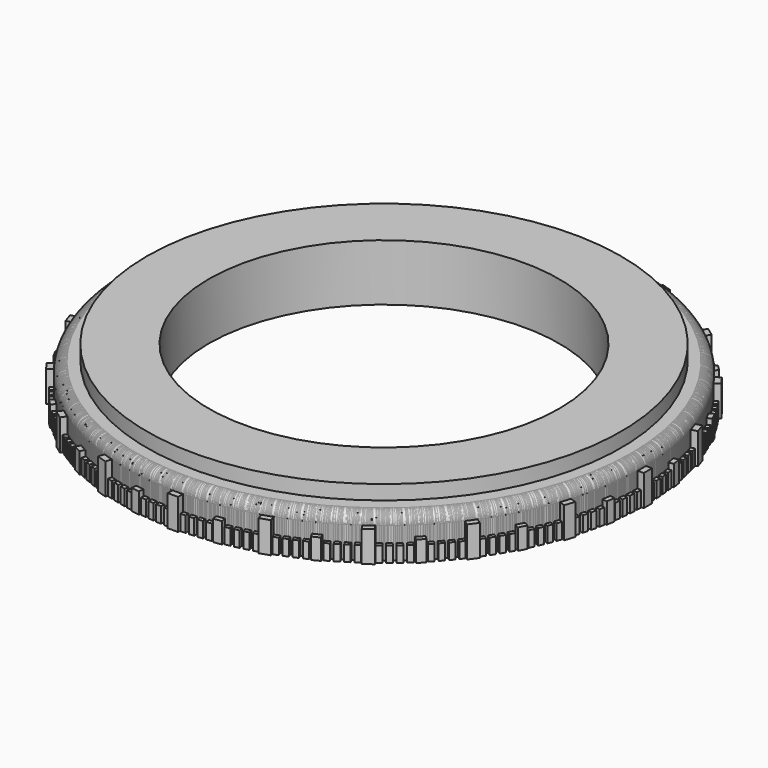
from build123d import *

# Parameters (mm, degrees)
F3_R      = 1
F4_W      = 1
F4_H      = 1
F5_DEPTH  = 3
F6_COUNT  = 20
F4_W_2    = 0.8
F4_H_2    = 0.8
F7_DEPTH  = 2
F8_COUNT  = 40
F4_W_3    = 0.5
F9_DEPTH  = 1.5
F10_COUNT = 200


with BuildPart() as f1:
    # F0 (on Front) → F1 (revolve)
    with BuildSketch(Plane.XZ):
        with BuildLine():
            Line((-20, 0), (-17, 0))
            Line((-17, 0), (-17, 4))
            Line((-17, 4), (-20, 4))
            add(Edge.make_bspline(
                [(-20, 4), (-20.2, 3.3333333333), (-20.6, 2), (-20.2, 0.6666666667), (-20, 0)],
                knots=[0, 0, 0, 0, 0.5, 1, 1, 1, 1], degree=3))
        make_face()
        Polygon((-20, 4), (-17, 4), (-17, 5.5), (-23, 5.5), (-23, 4.1), (-20, 4.1), align=None)
    revolve(axis=Axis((0, 0, 11.5319285542), (0, 0, 1)))


with BuildPart() as f2:
    # F0 (on Front) → F2 (revolve)
    with BuildSketch(Plane.XZ):
        with BuildLine():
            add(Edge.make_bspline(
                [(-20.25, 4), (-20.375, 3.3333333333), (-20.625, 2), (-20.375, 0.6666666667), (-20.25, 0)],
                knots=[0, 0, 0, 0, 0.5, 1, 1, 1, 1], degree=3))
            Line((-20.25, 4), (-25, 4))
            Line((-25, 4), (-25, 0))
            Line((-25, 0), (-20.25, 0))
        make_face()
    revolve(axis=Axis((0, 0, 11.5319285542), (0, 0, 1)))

    # F3
    f3_edges = [f2.edges().sort_by_distance(p)[0] for p in [
        (25, 0, 4),
    ]]
    fillet(f3_edges, radius=F3_R)

    # F4 (on Top) → F5 (join)
    with BuildSketch(Plane.XY):
        with Locations((-25.0881966203, 0)):
            Rectangle(F4_W, F4_H)
    extrude(amount=F5_DEPTH)


with BuildPart() as f6_1:
    # F6: instance of F2
    add(f2.part.rotate(Axis((0, 0, 11.5319285542), (0, 0, 1)), 1 * 360 / F6_COUNT))


with BuildPart() as f6_2:
    # F6: instance of F2
    add(f2.part.rotate(Axis((0, 0, 11.5319285542), (0, 0, 1)), 2 * 360 / F6_COUNT))


with BuildPart() as f6_3:
    # F6: instance of F2
    add(f2.part.rotate(Axis((0, 0, 11.5319285542), (0, 0, 1)), 3 * 360 / F6_COUNT))


with BuildPart() as f6_4:
    # F6: instance of F2
    add(f2.part.rotate(Axis((0, 0, 11.5319285542), (0, 0, 1)), 4 * 360 / F6_COUNT))


with BuildPart() as f6_5:
    # F6: instance of F2
    add(f2.part.rotate(Axis((0, 0, 11.5319285542), (0, 0, 1)), 5 * 360 / F6_COUNT))


with BuildPart() as f6_6:
    # F6: instance of F2
    add(f2.part.rotate(Axis((0, 0, 11.5319285542), (0, 0, 1)), 6 * 360 / F6_COUNT))


with BuildPart() as f6_7:
    # F6: instance of F2
    add(f2.part.rotate(Axis((0, 0, 11.5319285542), (0, 0, 1)), 7 * 360 / F6_COUNT))


with BuildPart() as f6_8:
    # F6: instance of F2
    add(f2.part.rotate(Axis((0, 0, 11.5319285542), (0, 0, 1)), 8 * 360 / F6_COUNT))


with BuildPart() as f6_9:
    # F6: instance of F2
    add(f2.part.rotate(Axis((0, 0, 11.5319285542), (0, 0, 1)), 9 * 360 / F6_COUNT))


with BuildPart() as f6_10:
    # F6: instance of F2
    add(f2.part.rotate(Axis((0, 0, 11.5319285542), (0, 0, 1)), 10 * 360 / F6_COUNT))


with BuildPart() as f6_11:
    # F6: instance of F2
    add(f2.part.rotate(Axis((0, 0, 11.5319285542), (0, 0, 1)), 11 * 360 / F6_COUNT))


with BuildPart() as f6_12:
    # F6: instance of F2
    add(f2.part.rotate(Axis((0, 0, 11.5319285542), (0, 0, 1)), 12 * 360 / F6_COUNT))


with BuildPart() as f6_13:
    # F6: instance of F2
    add(f2.part.rotate(Axis((0, 0, 11.5319285542), (0, 0, 1)), 13 * 360 / F6_COUNT))


with BuildPart() as f6_14:
    # F6: instance of F2
    add(f2.part.rotate(Axis((0, 0, 11.5319285542), (0, 0, 1)), 14 * 360 / F6_COUNT))


with BuildPart() as f6_15:
    # F6: instance of F2
    add(f2.part.rotate(Axis((0, 0, 11.5319285542), (0, 0, 1)), 15 * 360 / F6_COUNT))


with BuildPart() as f6_16:
    # F6: instance of F2
    add(f2.part.rotate(Axis((0, 0, 11.5319285542), (0, 0, 1)), 16 * 360 / F6_COUNT))


with BuildPart() as f6_17:
    # F6: instance of F2
    add(f2.part.rotate(Axis((0, 0, 11.5319285542), (0, 0, 1)), 17 * 360 / F6_COUNT))


with BuildPart() as f6_18:
    # F6: instance of F2
    add(f2.part.rotate(Axis((0, 0, 11.5319285542), (0, 0, 1)), 18 * 360 / F6_COUNT))


with BuildPart() as f6_19:
    # F6: instance of F2
    add(f2.part.rotate(Axis((0, 0, 11.5319285542), (0, 0, 1)), 19 * 360 / F6_COUNT))


with BuildPart() as f7:
    # F4 (on Top) → F7 (new body)
    with BuildSketch(Plane.XY):
        with Locations((25.0804126263, 0)):
            Rectangle(F4_W_2, F4_H_2)
    extrude(amount=F7_DEPTH)


with BuildPart() as f8_1:
    # F8: instance of F7
    add(f7.part.rotate(Axis((0, 0, 11.5319285542), (0, 0, 1)), 1 * 360 / F8_COUNT))


with BuildPart() as f8_2:
    # F8: instance of F7
    add(f7.part.rotate(Axis((0, 0, 11.5319285542), (0, 0, 1)), 2 * 360 / F8_COUNT))


with BuildPart() as f8_3:
    # F8: instance of F7
    add(f7.part.rotate(Axis((0, 0, 11.5319285542), (0, 0, 1)), 3 * 360 / F8_COUNT))


with BuildPart() as f8_4:
    # F8: instance of F7
    add(f7.part.rotate(Axis((0, 0, 11.5319285542), (0, 0, 1)), 4 * 360 / F8_COUNT))


with BuildPart() as f8_5:
    # F8: instance of F7
    add(f7.part.rotate(Axis((0, 0, 11.5319285542), (0, 0, 1)), 5 * 360 / F8_COUNT))


with BuildPart() as f8_6:
    # F8: instance of F7
    add(f7.part.rotate(Axis((0, 0, 11.5319285542), (0, 0, 1)), 6 * 360 / F8_COUNT))


with BuildPart() as f8_7:
    # F8: instance of F7
    add(f7.part.rotate(Axis((0, 0, 11.5319285542), (0, 0, 1)), 7 * 360 / F8_COUNT))


with BuildPart() as f8_8:
    # F8: instance of F7
    add(f7.part.rotate(Axis((0, 0, 11.5319285542), (0, 0, 1)), 8 * 360 / F8_COUNT))


with BuildPart() as f8_9:
    # F8: instance of F7
    add(f7.part.rotate(Axis((0, 0, 11.5319285542), (0, 0, 1)), 9 * 360 / F8_COUNT))


with BuildPart() as f8_10:
    # F8: instance of F7
    add(f7.part.rotate(Axis((0, 0, 11.5319285542), (0, 0, 1)), 10 * 360 / F8_COUNT))


with BuildPart() as f8_11:
    # F8: instance of F7
    add(f7.part.rotate(Axis((0, 0, 11.5319285542), (0, 0, 1)), 11 * 360 / F8_COUNT))


with BuildPart() as f8_12:
    # F8: instance of F7
    add(f7.part.rotate(Axis((0, 0, 11.5319285542), (0, 0, 1)), 12 * 360 / F8_COUNT))


with BuildPart() as f8_13:
    # F8: instance of F7
    add(f7.part.rotate(Axis((0, 0, 11.5319285542), (0, 0, 1)), 13 * 360 / F8_COUNT))


with BuildPart() as f8_14:
    # F8: instance of F7
    add(f7.part.rotate(Axis((0, 0, 11.5319285542), (0, 0, 1)), 14 * 360 / F8_COUNT))


with BuildPart() as f8_15:
    # F8: instance of F7
    add(f7.part.rotate(Axis((0, 0, 11.5319285542), (0, 0, 1)), 15 * 360 / F8_COUNT))


with BuildPart() as f8_16:
    # F8: instance of F7
    add(f7.part.rotate(Axis((0, 0, 11.5319285542), (0, 0, 1)), 16 * 360 / F8_COUNT))


with BuildPart() as f8_17:
    # F8: instance of F7
    add(f7.part.rotate(Axis((0, 0, 11.5319285542), (0, 0, 1)), 17 * 360 / F8_COUNT))


with BuildPart() as f8_18:
    # F8: instance of F7
    add(f7.part.rotate(Axis((0, 0, 11.5319285542), (0, 0, 1)), 18 * 360 / F8_COUNT))


with BuildPart() as f8_19:
    # F8: instance of F7
    add(f7.part.rotate(Axis((0, 0, 11.5319285542), (0, 0, 1)), 19 * 360 / F8_COUNT))


with BuildPart() as f8_20:
    # F8: instance of F7
    add(f7.part.rotate(Axis((0, 0, 11.5319285542), (0, 0, 1)), 20 * 360 / F8_COUNT))


with BuildPart() as f8_21:
    # F8: instance of F7
    add(f7.part.rotate(Axis((0, 0, 11.5319285542), (0, 0, 1)), 21 * 360 / F8_COUNT))


with BuildPart() as f8_22:
    # F8: instance of F7
    add(f7.part.rotate(Axis((0, 0, 11.5319285542), (0, 0, 1)), 22 * 360 / F8_COUNT))


with BuildPart() as f8_23:
    # F8: instance of F7
    add(f7.part.rotate(Axis((0, 0, 11.5319285542), (0, 0, 1)), 23 * 360 / F8_COUNT))


with BuildPart() as f8_24:
    # F8: instance of F7
    add(f7.part.rotate(Axis((0, 0, 11.5319285542), (0, 0, 1)), 24 * 360 / F8_COUNT))


with BuildPart() as f8_25:
    # F8: instance of F7
    add(f7.part.rotate(Axis((0, 0, 11.5319285542), (0, 0, 1)), 25 * 360 / F8_COUNT))


with BuildPart() as f8_26:
    # F8: instance of F7
    add(f7.part.rotate(Axis((0, 0, 11.5319285542), (0, 0, 1)), 26 * 360 / F8_COUNT))


with BuildPart() as f8_27:
    # F8: instance of F7
    add(f7.part.rotate(Axis((0, 0, 11.5319285542), (0, 0, 1)), 27 * 360 / F8_COUNT))


with BuildPart() as f8_28:
    # F8: instance of F7
    add(f7.part.rotate(Axis((0, 0, 11.5319285542), (0, 0, 1)), 28 * 360 / F8_COUNT))


with BuildPart() as f8_29:
    # F8: instance of F7
    add(f7.part.rotate(Axis((0, 0, 11.5319285542), (0, 0, 1)), 29 * 360 / F8_COUNT))


with BuildPart() as f8_30:
    # F8: instance of F7
    add(f7.part.rotate(Axis((0, 0, 11.5319285542), (0, 0, 1)), 30 * 360 / F8_COUNT))


with BuildPart() as f8_31:
    # F8: instance of F7
    add(f7.part.rotate(Axis((0, 0, 11.5319285542), (0, 0, 1)), 31 * 360 / F8_COUNT))


with BuildPart() as f8_32:
    # F8: instance of F7
    add(f7.part.rotate(Axis((0, 0, 11.5319285542), (0, 0, 1)), 32 * 360 / F8_COUNT))


with BuildPart() as f8_33:
    # F8: instance of F7
    add(f7.part.rotate(Axis((0, 0, 11.5319285542), (0, 0, 1)), 33 * 360 / F8_COUNT))


with BuildPart() as f8_34:
    # F8: instance of F7
    add(f7.part.rotate(Axis((0, 0, 11.5319285542), (0, 0, 1)), 34 * 360 / F8_COUNT))


with BuildPart() as f8_35:
    # F8: instance of F7
    add(f7.part.rotate(Axis((0, 0, 11.5319285542), (0, 0, 1)), 35 * 360 / F8_COUNT))


with BuildPart() as f8_36:
    # F8: instance of F7
    add(f7.part.rotate(Axis((0, 0, 11.5319285542), (0, 0, 1)), 36 * 360 / F8_COUNT))


with BuildPart() as f8_37:
    # F8: instance of F7
    add(f7.part.rotate(Axis((0, 0, 11.5319285542), (0, 0, 1)), 37 * 360 / F8_COUNT))


with BuildPart() as f8_38:
    # F8: instance of F7
    add(f7.part.rotate(Axis((0, 0, 11.5319285542), (0, 0, 1)), 38 * 360 / F8_COUNT))


with BuildPart() as f8_39:
    # F8: instance of F7
    add(f7.part.rotate(Axis((0, 0, 11.5319285542), (0, 0, 1)), 39 * 360 / F8_COUNT))


with BuildPart() as f9:
    # F4 (on Top) → F9 (new body)
    with BuildSketch(Plane.XY):
        with Locations((0, -24.9772239476)):
            Rectangle(F4_W_3, F4_H_2)
    extrude(amount=F9_DEPTH)


with BuildPart() as f10_1:
    # F10: instance of F9
    add(f9.part.rotate(Axis((0, 0, 11.5319285542), (0, 0, 1)), 1 * 360 / F10_COUNT))


with BuildPart() as f10_2:
    # F10: instance of F9
    add(f9.part.rotate(Axis((0, 0, 11.5319285542), (0, 0, 1)), 2 * 360 / F10_COUNT))


with BuildPart() as f10_3:
    # F10: instance of F9
    add(f9.part.rotate(Axis((0, 0, 11.5319285542), (0, 0, 1)), 3 * 360 / F10_COUNT))


with BuildPart() as f10_4:
    # F10: instance of F9
    add(f9.part.rotate(Axis((0, 0, 11.5319285542), (0, 0, 1)), 4 * 360 / F10_COUNT))


with BuildPart() as f10_5:
    # F10: instance of F9
    add(f9.part.rotate(Axis((0, 0, 11.5319285542), (0, 0, 1)), 5 * 360 / F10_COUNT))


with BuildPart() as f10_6:
    # F10: instance of F9
    add(f9.part.rotate(Axis((0, 0, 11.5319285542), (0, 0, 1)), 6 * 360 / F10_COUNT))


with BuildPart() as f10_7:
    # F10: instance of F9
    add(f9.part.rotate(Axis((0, 0, 11.5319285542), (0, 0, 1)), 7 * 360 / F10_COUNT))


with BuildPart() as f10_8:
    # F10: instance of F9
    add(f9.part.rotate(Axis((0, 0, 11.5319285542), (0, 0, 1)), 8 * 360 / F10_COUNT))


with BuildPart() as f10_9:
    # F10: instance of F9
    add(f9.part.rotate(Axis((0, 0, 11.5319285542), (0, 0, 1)), 9 * 360 / F10_COUNT))


with BuildPart() as f10_10:
    # F10: instance of F9
    add(f9.part.rotate(Axis((0, 0, 11.5319285542), (0, 0, 1)), 10 * 360 / F10_COUNT))


with BuildPart() as f10_11:
    # F10: instance of F9
    add(f9.part.rotate(Axis((0, 0, 11.5319285542), (0, 0, 1)), 11 * 360 / F10_COUNT))


with BuildPart() as f10_12:
    # F10: instance of F9
    add(f9.part.rotate(Axis((0, 0, 11.5319285542), (0, 0, 1)), 12 * 360 / F10_COUNT))


with BuildPart() as f10_13:
    # F10: instance of F9
    add(f9.part.rotate(Axis((0, 0, 11.5319285542), (0, 0, 1)), 13 * 360 / F10_COUNT))


with BuildPart() as f10_14:
    # F10: instance of F9
    add(f9.part.rotate(Axis((0, 0, 11.5319285542), (0, 0, 1)), 14 * 360 / F10_COUNT))


with BuildPart() as f10_15:
    # F10: instance of F9
    add(f9.part.rotate(Axis((0, 0, 11.5319285542), (0, 0, 1)), 15 * 360 / F10_COUNT))


with BuildPart() as f10_16:
    # F10: instance of F9
    add(f9.part.rotate(Axis((0, 0, 11.5319285542), (0, 0, 1)), 16 * 360 / F10_COUNT))


with BuildPart() as f10_17:
    # F10: instance of F9
    add(f9.part.rotate(Axis((0, 0, 11.5319285542), (0, 0, 1)), 17 * 360 / F10_COUNT))


with BuildPart() as f10_18:
    # F10: instance of F9
    add(f9.part.rotate(Axis((0, 0, 11.5319285542), (0, 0, 1)), 18 * 360 / F10_COUNT))


with BuildPart() as f10_19:
    # F10: instance of F9
    add(f9.part.rotate(Axis((0, 0, 11.5319285542), (0, 0, 1)), 19 * 360 / F10_COUNT))


with BuildPart() as f10_20:
    # F10: instance of F9
    add(f9.part.rotate(Axis((0, 0, 11.5319285542), (0, 0, 1)), 20 * 360 / F10_COUNT))


with BuildPart() as f10_21:
    # F10: instance of F9
    add(f9.part.rotate(Axis((0, 0, 11.5319285542), (0, 0, 1)), 21 * 360 / F10_COUNT))


with BuildPart() as f10_22:
    # F10: instance of F9
    add(f9.part.rotate(Axis((0, 0, 11.5319285542), (0, 0, 1)), 22 * 360 / F10_COUNT))


with BuildPart() as f10_23:
    # F10: instance of F9
    add(f9.part.rotate(Axis((0, 0, 11.5319285542), (0, 0, 1)), 23 * 360 / F10_COUNT))


with BuildPart() as f10_24:
    # F10: instance of F9
    add(f9.part.rotate(Axis((0, 0, 11.5319285542), (0, 0, 1)), 24 * 360 / F10_COUNT))


with BuildPart() as f10_25:
    # F10: instance of F9
    add(f9.part.rotate(Axis((0, 0, 11.5319285542), (0, 0, 1)), 25 * 360 / F10_COUNT))


with BuildPart() as f10_26:
    # F10: instance of F9
    add(f9.part.rotate(Axis((0, 0, 11.5319285542), (0, 0, 1)), 26 * 360 / F10_COUNT))


with BuildPart() as f10_27:
    # F10: instance of F9
    add(f9.part.rotate(Axis((0, 0, 11.5319285542), (0, 0, 1)), 27 * 360 / F10_COUNT))


with BuildPart() as f10_28:
    # F10: instance of F9
    add(f9.part.rotate(Axis((0, 0, 11.5319285542), (0, 0, 1)), 28 * 360 / F10_COUNT))


with BuildPart() as f10_29:
    # F10: instance of F9
    add(f9.part.rotate(Axis((0, 0, 11.5319285542), (0, 0, 1)), 29 * 360 / F10_COUNT))


with BuildPart() as f10_30:
    # F10: instance of F9
    add(f9.part.rotate(Axis((0, 0, 11.5319285542), (0, 0, 1)), 30 * 360 / F10_COUNT))


with BuildPart() as f10_31:
    # F10: instance of F9
    add(f9.part.rotate(Axis((0, 0, 11.5319285542), (0, 0, 1)), 31 * 360 / F10_COUNT))


with BuildPart() as f10_32:
    # F10: instance of F9
    add(f9.part.rotate(Axis((0, 0, 11.5319285542), (0, 0, 1)), 32 * 360 / F10_COUNT))


with BuildPart() as f10_33:
    # F10: instance of F9
    add(f9.part.rotate(Axis((0, 0, 11.5319285542), (0, 0, 1)), 33 * 360 / F10_COUNT))


with BuildPart() as f10_34:
    # F10: instance of F9
    add(f9.part.rotate(Axis((0, 0, 11.5319285542), (0, 0, 1)), 34 * 360 / F10_COUNT))


with BuildPart() as f10_35:
    # F10: instance of F9
    add(f9.part.rotate(Axis((0, 0, 11.5319285542), (0, 0, 1)), 35 * 360 / F10_COUNT))


with BuildPart() as f10_36:
    # F10: instance of F9
    add(f9.part.rotate(Axis((0, 0, 11.5319285542), (0, 0, 1)), 36 * 360 / F10_COUNT))


with BuildPart() as f10_37:
    # F10: instance of F9
    add(f9.part.rotate(Axis((0, 0, 11.5319285542), (0, 0, 1)), 37 * 360 / F10_COUNT))


with BuildPart() as f10_38:
    # F10: instance of F9
    add(f9.part.rotate(Axis((0, 0, 11.5319285542), (0, 0, 1)), 38 * 360 / F10_COUNT))


with BuildPart() as f10_39:
    # F10: instance of F9
    add(f9.part.rotate(Axis((0, 0, 11.5319285542), (0, 0, 1)), 39 * 360 / F10_COUNT))


with BuildPart() as f10_40:
    # F10: instance of F9
    add(f9.part.rotate(Axis((0, 0, 11.5319285542), (0, 0, 1)), 40 * 360 / F10_COUNT))


with BuildPart() as f10_41:
    # F10: instance of F9
    add(f9.part.rotate(Axis((0, 0, 11.5319285542), (0, 0, 1)), 41 * 360 / F10_COUNT))


with BuildPart() as f10_42:
    # F10: instance of F9
    add(f9.part.rotate(Axis((0, 0, 11.5319285542), (0, 0, 1)), 42 * 360 / F10_COUNT))


with BuildPart() as f10_43:
    # F10: instance of F9
    add(f9.part.rotate(Axis((0, 0, 11.5319285542), (0, 0, 1)), 43 * 360 / F10_COUNT))


with BuildPart() as f10_44:
    # F10: instance of F9
    add(f9.part.rotate(Axis((0, 0, 11.5319285542), (0, 0, 1)), 44 * 360 / F10_COUNT))


with BuildPart() as f10_45:
    # F10: instance of F9
    add(f9.part.rotate(Axis((0, 0, 11.5319285542), (0, 0, 1)), 45 * 360 / F10_COUNT))


with BuildPart() as f10_46:
    # F10: instance of F9
    add(f9.part.rotate(Axis((0, 0, 11.5319285542), (0, 0, 1)), 46 * 360 / F10_COUNT))


with BuildPart() as f10_47:
    # F10: instance of F9
    add(f9.part.rotate(Axis((0, 0, 11.5319285542), (0, 0, 1)), 47 * 360 / F10_COUNT))


with BuildPart() as f10_48:
    # F10: instance of F9
    add(f9.part.rotate(Axis((0, 0, 11.5319285542), (0, 0, 1)), 48 * 360 / F10_COUNT))


with BuildPart() as f10_49:
    # F10: instance of F9
    add(f9.part.rotate(Axis((0, 0, 11.5319285542), (0, 0, 1)), 49 * 360 / F10_COUNT))


with BuildPart() as f10_50:
    # F10: instance of F9
    add(f9.part.rotate(Axis((0, 0, 11.5319285542), (0, 0, 1)), 50 * 360 / F10_COUNT))


with BuildPart() as f10_51:
    # F10: instance of F9
    add(f9.part.rotate(Axis((0, 0, 11.5319285542), (0, 0, 1)), 51 * 360 / F10_COUNT))


with BuildPart() as f10_52:
    # F10: instance of F9
    add(f9.part.rotate(Axis((0, 0, 11.5319285542), (0, 0, 1)), 52 * 360 / F10_COUNT))


with BuildPart() as f10_53:
    # F10: instance of F9
    add(f9.part.rotate(Axis((0, 0, 11.5319285542), (0, 0, 1)), 53 * 360 / F10_COUNT))


with BuildPart() as f10_54:
    # F10: instance of F9
    add(f9.part.rotate(Axis((0, 0, 11.5319285542), (0, 0, 1)), 54 * 360 / F10_COUNT))


with BuildPart() as f10_55:
    # F10: instance of F9
    add(f9.part.rotate(Axis((0, 0, 11.5319285542), (0, 0, 1)), 55 * 360 / F10_COUNT))


with BuildPart() as f10_56:
    # F10: instance of F9
    add(f9.part.rotate(Axis((0, 0, 11.5319285542), (0, 0, 1)), 56 * 360 / F10_COUNT))


with BuildPart() as f10_57:
    # F10: instance of F9
    add(f9.part.rotate(Axis((0, 0, 11.5319285542), (0, 0, 1)), 57 * 360 / F10_COUNT))


with BuildPart() as f10_58:
    # F10: instance of F9
    add(f9.part.rotate(Axis((0, 0, 11.5319285542), (0, 0, 1)), 58 * 360 / F10_COUNT))


with BuildPart() as f10_59:
    # F10: instance of F9
    add(f9.part.rotate(Axis((0, 0, 11.5319285542), (0, 0, 1)), 59 * 360 / F10_COUNT))


with BuildPart() as f10_60:
    # F10: instance of F9
    add(f9.part.rotate(Axis((0, 0, 11.5319285542), (0, 0, 1)), 60 * 360 / F10_COUNT))


with BuildPart() as f10_61:
    # F10: instance of F9
    add(f9.part.rotate(Axis((0, 0, 11.5319285542), (0, 0, 1)), 61 * 360 / F10_COUNT))


with BuildPart() as f10_62:
    # F10: instance of F9
    add(f9.part.rotate(Axis((0, 0, 11.5319285542), (0, 0, 1)), 62 * 360 / F10_COUNT))


with BuildPart() as f10_63:
    # F10: instance of F9
    add(f9.part.rotate(Axis((0, 0, 11.5319285542), (0, 0, 1)), 63 * 360 / F10_COUNT))


with BuildPart() as f10_64:
    # F10: instance of F9
    add(f9.part.rotate(Axis((0, 0, 11.5319285542), (0, 0, 1)), 64 * 360 / F10_COUNT))


with BuildPart() as f10_65:
    # F10: instance of F9
    add(f9.part.rotate(Axis((0, 0, 11.5319285542), (0, 0, 1)), 65 * 360 / F10_COUNT))


with BuildPart() as f10_66:
    # F10: instance of F9
    add(f9.part.rotate(Axis((0, 0, 11.5319285542), (0, 0, 1)), 66 * 360 / F10_COUNT))


with BuildPart() as f10_67:
    # F10: instance of F9
    add(f9.part.rotate(Axis((0, 0, 11.5319285542), (0, 0, 1)), 67 * 360 / F10_COUNT))


with BuildPart() as f10_68:
    # F10: instance of F9
    add(f9.part.rotate(Axis((0, 0, 11.5319285542), (0, 0, 1)), 68 * 360 / F10_COUNT))


with BuildPart() as f10_69:
    # F10: instance of F9
    add(f9.part.rotate(Axis((0, 0, 11.5319285542), (0, 0, 1)), 69 * 360 / F10_COUNT))


with BuildPart() as f10_70:
    # F10: instance of F9
    add(f9.part.rotate(Axis((0, 0, 11.5319285542), (0, 0, 1)), 70 * 360 / F10_COUNT))


with BuildPart() as f10_71:
    # F10: instance of F9
    add(f9.part.rotate(Axis((0, 0, 11.5319285542), (0, 0, 1)), 71 * 360 / F10_COUNT))


with BuildPart() as f10_72:
    # F10: instance of F9
    add(f9.part.rotate(Axis((0, 0, 11.5319285542), (0, 0, 1)), 72 * 360 / F10_COUNT))


with BuildPart() as f10_73:
    # F10: instance of F9
    add(f9.part.rotate(Axis((0, 0, 11.5319285542), (0, 0, 1)), 73 * 360 / F10_COUNT))


with BuildPart() as f10_74:
    # F10: instance of F9
    add(f9.part.rotate(Axis((0, 0, 11.5319285542), (0, 0, 1)), 74 * 360 / F10_COUNT))


with BuildPart() as f10_75:
    # F10: instance of F9
    add(f9.part.rotate(Axis((0, 0, 11.5319285542), (0, 0, 1)), 75 * 360 / F10_COUNT))


with BuildPart() as f10_76:
    # F10: instance of F9
    add(f9.part.rotate(Axis((0, 0, 11.5319285542), (0, 0, 1)), 76 * 360 / F10_COUNT))


with BuildPart() as f10_77:
    # F10: instance of F9
    add(f9.part.rotate(Axis((0, 0, 11.5319285542), (0, 0, 1)), 77 * 360 / F10_COUNT))


with BuildPart() as f10_78:
    # F10: instance of F9
    add(f9.part.rotate(Axis((0, 0, 11.5319285542), (0, 0, 1)), 78 * 360 / F10_COUNT))


with BuildPart() as f10_79:
    # F10: instance of F9
    add(f9.part.rotate(Axis((0, 0, 11.5319285542), (0, 0, 1)), 79 * 360 / F10_COUNT))


with BuildPart() as f10_80:
    # F10: instance of F9
    add(f9.part.rotate(Axis((0, 0, 11.5319285542), (0, 0, 1)), 80 * 360 / F10_COUNT))


with BuildPart() as f10_81:
    # F10: instance of F9
    add(f9.part.rotate(Axis((0, 0, 11.5319285542), (0, 0, 1)), 81 * 360 / F10_COUNT))


with BuildPart() as f10_82:
    # F10: instance of F9
    add(f9.part.rotate(Axis((0, 0, 11.5319285542), (0, 0, 1)), 82 * 360 / F10_COUNT))


with BuildPart() as f10_83:
    # F10: instance of F9
    add(f9.part.rotate(Axis((0, 0, 11.5319285542), (0, 0, 1)), 83 * 360 / F10_COUNT))


with BuildPart() as f10_84:
    # F10: instance of F9
    add(f9.part.rotate(Axis((0, 0, 11.5319285542), (0, 0, 1)), 84 * 360 / F10_COUNT))


with BuildPart() as f10_85:
    # F10: instance of F9
    add(f9.part.rotate(Axis((0, 0, 11.5319285542), (0, 0, 1)), 85 * 360 / F10_COUNT))


with BuildPart() as f10_86:
    # F10: instance of F9
    add(f9.part.rotate(Axis((0, 0, 11.5319285542), (0, 0, 1)), 86 * 360 / F10_COUNT))


with BuildPart() as f10_87:
    # F10: instance of F9
    add(f9.part.rotate(Axis((0, 0, 11.5319285542), (0, 0, 1)), 87 * 360 / F10_COUNT))


with BuildPart() as f10_88:
    # F10: instance of F9
    add(f9.part.rotate(Axis((0, 0, 11.5319285542), (0, 0, 1)), 88 * 360 / F10_COUNT))


with BuildPart() as f10_89:
    # F10: instance of F9
    add(f9.part.rotate(Axis((0, 0, 11.5319285542), (0, 0, 1)), 89 * 360 / F10_COUNT))


with BuildPart() as f10_90:
    # F10: instance of F9
    add(f9.part.rotate(Axis((0, 0, 11.5319285542), (0, 0, 1)), 90 * 360 / F10_COUNT))


with BuildPart() as f10_91:
    # F10: instance of F9
    add(f9.part.rotate(Axis((0, 0, 11.5319285542), (0, 0, 1)), 91 * 360 / F10_COUNT))


with BuildPart() as f10_92:
    # F10: instance of F9
    add(f9.part.rotate(Axis((0, 0, 11.5319285542), (0, 0, 1)), 92 * 360 / F10_COUNT))


with BuildPart() as f10_93:
    # F10: instance of F9
    add(f9.part.rotate(Axis((0, 0, 11.5319285542), (0, 0, 1)), 93 * 360 / F10_COUNT))


with BuildPart() as f10_94:
    # F10: instance of F9
    add(f9.part.rotate(Axis((0, 0, 11.5319285542), (0, 0, 1)), 94 * 360 / F10_COUNT))


with BuildPart() as f10_95:
    # F10: instance of F9
    add(f9.part.rotate(Axis((0, 0, 11.5319285542), (0, 0, 1)), 95 * 360 / F10_COUNT))


with BuildPart() as f10_96:
    # F10: instance of F9
    add(f9.part.rotate(Axis((0, 0, 11.5319285542), (0, 0, 1)), 96 * 360 / F10_COUNT))


with BuildPart() as f10_97:
    # F10: instance of F9
    add(f9.part.rotate(Axis((0, 0, 11.5319285542), (0, 0, 1)), 97 * 360 / F10_COUNT))


with BuildPart() as f10_98:
    # F10: instance of F9
    add(f9.part.rotate(Axis((0, 0, 11.5319285542), (0, 0, 1)), 98 * 360 / F10_COUNT))


with BuildPart() as f10_99:
    # F10: instance of F9
    add(f9.part.rotate(Axis((0, 0, 11.5319285542), (0, 0, 1)), 99 * 360 / F10_COUNT))


with BuildPart() as f10_100:
    # F10: instance of F9
    add(f9.part.rotate(Axis((0, 0, 11.5319285542), (0, 0, 1)), 100 * 360 / F10_COUNT))


with BuildPart() as f10_101:
    # F10: instance of F9
    add(f9.part.rotate(Axis((0, 0, 11.5319285542), (0, 0, 1)), 101 * 360 / F10_COUNT))


with BuildPart() as f10_102:
    # F10: instance of F9
    add(f9.part.rotate(Axis((0, 0, 11.5319285542), (0, 0, 1)), 102 * 360 / F10_COUNT))


with BuildPart() as f10_103:
    # F10: instance of F9
    add(f9.part.rotate(Axis((0, 0, 11.5319285542), (0, 0, 1)), 103 * 360 / F10_COUNT))


with BuildPart() as f10_104:
    # F10: instance of F9
    add(f9.part.rotate(Axis((0, 0, 11.5319285542), (0, 0, 1)), 104 * 360 / F10_COUNT))


with BuildPart() as f10_105:
    # F10: instance of F9
    add(f9.part.rotate(Axis((0, 0, 11.5319285542), (0, 0, 1)), 105 * 360 / F10_COUNT))


with BuildPart() as f10_106:
    # F10: instance of F9
    add(f9.part.rotate(Axis((0, 0, 11.5319285542), (0, 0, 1)), 106 * 360 / F10_COUNT))


with BuildPart() as f10_107:
    # F10: instance of F9
    add(f9.part.rotate(Axis((0, 0, 11.5319285542), (0, 0, 1)), 107 * 360 / F10_COUNT))


with BuildPart() as f10_108:
    # F10: instance of F9
    add(f9.part.rotate(Axis((0, 0, 11.5319285542), (0, 0, 1)), 108 * 360 / F10_COUNT))


with BuildPart() as f10_109:
    # F10: instance of F9
    add(f9.part.rotate(Axis((0, 0, 11.5319285542), (0, 0, 1)), 109 * 360 / F10_COUNT))


with BuildPart() as f10_110:
    # F10: instance of F9
    add(f9.part.rotate(Axis((0, 0, 11.5319285542), (0, 0, 1)), 110 * 360 / F10_COUNT))


with BuildPart() as f10_111:
    # F10: instance of F9
    add(f9.part.rotate(Axis((0, 0, 11.5319285542), (0, 0, 1)), 111 * 360 / F10_COUNT))


with BuildPart() as f10_112:
    # F10: instance of F9
    add(f9.part.rotate(Axis((0, 0, 11.5319285542), (0, 0, 1)), 112 * 360 / F10_COUNT))


with BuildPart() as f10_113:
    # F10: instance of F9
    add(f9.part.rotate(Axis((0, 0, 11.5319285542), (0, 0, 1)), 113 * 360 / F10_COUNT))


with BuildPart() as f10_114:
    # F10: instance of F9
    add(f9.part.rotate(Axis((0, 0, 11.5319285542), (0, 0, 1)), 114 * 360 / F10_COUNT))


with BuildPart() as f10_115:
    # F10: instance of F9
    add(f9.part.rotate(Axis((0, 0, 11.5319285542), (0, 0, 1)), 115 * 360 / F10_COUNT))


with BuildPart() as f10_116:
    # F10: instance of F9
    add(f9.part.rotate(Axis((0, 0, 11.5319285542), (0, 0, 1)), 116 * 360 / F10_COUNT))


with BuildPart() as f10_117:
    # F10: instance of F9
    add(f9.part.rotate(Axis((0, 0, 11.5319285542), (0, 0, 1)), 117 * 360 / F10_COUNT))


with BuildPart() as f10_118:
    # F10: instance of F9
    add(f9.part.rotate(Axis((0, 0, 11.5319285542), (0, 0, 1)), 118 * 360 / F10_COUNT))


with BuildPart() as f10_119:
    # F10: instance of F9
    add(f9.part.rotate(Axis((0, 0, 11.5319285542), (0, 0, 1)), 119 * 360 / F10_COUNT))


with BuildPart() as f10_120:
    # F10: instance of F9
    add(f9.part.rotate(Axis((0, 0, 11.5319285542), (0, 0, 1)), 120 * 360 / F10_COUNT))


with BuildPart() as f10_121:
    # F10: instance of F9
    add(f9.part.rotate(Axis((0, 0, 11.5319285542), (0, 0, 1)), 121 * 360 / F10_COUNT))


with BuildPart() as f10_122:
    # F10: instance of F9
    add(f9.part.rotate(Axis((0, 0, 11.5319285542), (0, 0, 1)), 122 * 360 / F10_COUNT))


with BuildPart() as f10_123:
    # F10: instance of F9
    add(f9.part.rotate(Axis((0, 0, 11.5319285542), (0, 0, 1)), 123 * 360 / F10_COUNT))


with BuildPart() as f10_124:
    # F10: instance of F9
    add(f9.part.rotate(Axis((0, 0, 11.5319285542), (0, 0, 1)), 124 * 360 / F10_COUNT))


with BuildPart() as f10_125:
    # F10: instance of F9
    add(f9.part.rotate(Axis((0, 0, 11.5319285542), (0, 0, 1)), 125 * 360 / F10_COUNT))


with BuildPart() as f10_126:
    # F10: instance of F9
    add(f9.part.rotate(Axis((0, 0, 11.5319285542), (0, 0, 1)), 126 * 360 / F10_COUNT))


with BuildPart() as f10_127:
    # F10: instance of F9
    add(f9.part.rotate(Axis((0, 0, 11.5319285542), (0, 0, 1)), 127 * 360 / F10_COUNT))


with BuildPart() as f10_128:
    # F10: instance of F9
    add(f9.part.rotate(Axis((0, 0, 11.5319285542), (0, 0, 1)), 128 * 360 / F10_COUNT))


with BuildPart() as f10_129:
    # F10: instance of F9
    add(f9.part.rotate(Axis((0, 0, 11.5319285542), (0, 0, 1)), 129 * 360 / F10_COUNT))


with BuildPart() as f10_130:
    # F10: instance of F9
    add(f9.part.rotate(Axis((0, 0, 11.5319285542), (0, 0, 1)), 130 * 360 / F10_COUNT))


with BuildPart() as f10_131:
    # F10: instance of F9
    add(f9.part.rotate(Axis((0, 0, 11.5319285542), (0, 0, 1)), 131 * 360 / F10_COUNT))


with BuildPart() as f10_132:
    # F10: instance of F9
    add(f9.part.rotate(Axis((0, 0, 11.5319285542), (0, 0, 1)), 132 * 360 / F10_COUNT))


with BuildPart() as f10_133:
    # F10: instance of F9
    add(f9.part.rotate(Axis((0, 0, 11.5319285542), (0, 0, 1)), 133 * 360 / F10_COUNT))


with BuildPart() as f10_134:
    # F10: instance of F9
    add(f9.part.rotate(Axis((0, 0, 11.5319285542), (0, 0, 1)), 134 * 360 / F10_COUNT))


with BuildPart() as f10_135:
    # F10: instance of F9
    add(f9.part.rotate(Axis((0, 0, 11.5319285542), (0, 0, 1)), 135 * 360 / F10_COUNT))


with BuildPart() as f10_136:
    # F10: instance of F9
    add(f9.part.rotate(Axis((0, 0, 11.5319285542), (0, 0, 1)), 136 * 360 / F10_COUNT))


with BuildPart() as f10_137:
    # F10: instance of F9
    add(f9.part.rotate(Axis((0, 0, 11.5319285542), (0, 0, 1)), 137 * 360 / F10_COUNT))


with BuildPart() as f10_138:
    # F10: instance of F9
    add(f9.part.rotate(Axis((0, 0, 11.5319285542), (0, 0, 1)), 138 * 360 / F10_COUNT))


with BuildPart() as f10_139:
    # F10: instance of F9
    add(f9.part.rotate(Axis((0, 0, 11.5319285542), (0, 0, 1)), 139 * 360 / F10_COUNT))


with BuildPart() as f10_140:
    # F10: instance of F9
    add(f9.part.rotate(Axis((0, 0, 11.5319285542), (0, 0, 1)), 140 * 360 / F10_COUNT))


with BuildPart() as f10_141:
    # F10: instance of F9
    add(f9.part.rotate(Axis((0, 0, 11.5319285542), (0, 0, 1)), 141 * 360 / F10_COUNT))


with BuildPart() as f10_142:
    # F10: instance of F9
    add(f9.part.rotate(Axis((0, 0, 11.5319285542), (0, 0, 1)), 142 * 360 / F10_COUNT))


with BuildPart() as f10_143:
    # F10: instance of F9
    add(f9.part.rotate(Axis((0, 0, 11.5319285542), (0, 0, 1)), 143 * 360 / F10_COUNT))


with BuildPart() as f10_144:
    # F10: instance of F9
    add(f9.part.rotate(Axis((0, 0, 11.5319285542), (0, 0, 1)), 144 * 360 / F10_COUNT))


with BuildPart() as f10_145:
    # F10: instance of F9
    add(f9.part.rotate(Axis((0, 0, 11.5319285542), (0, 0, 1)), 145 * 360 / F10_COUNT))


with BuildPart() as f10_146:
    # F10: instance of F9
    add(f9.part.rotate(Axis((0, 0, 11.5319285542), (0, 0, 1)), 146 * 360 / F10_COUNT))


with BuildPart() as f10_147:
    # F10: instance of F9
    add(f9.part.rotate(Axis((0, 0, 11.5319285542), (0, 0, 1)), 147 * 360 / F10_COUNT))


with BuildPart() as f10_148:
    # F10: instance of F9
    add(f9.part.rotate(Axis((0, 0, 11.5319285542), (0, 0, 1)), 148 * 360 / F10_COUNT))


with BuildPart() as f10_149:
    # F10: instance of F9
    add(f9.part.rotate(Axis((0, 0, 11.5319285542), (0, 0, 1)), 149 * 360 / F10_COUNT))


with BuildPart() as f10_150:
    # F10: instance of F9
    add(f9.part.rotate(Axis((0, 0, 11.5319285542), (0, 0, 1)), 150 * 360 / F10_COUNT))


with BuildPart() as f10_151:
    # F10: instance of F9
    add(f9.part.rotate(Axis((0, 0, 11.5319285542), (0, 0, 1)), 151 * 360 / F10_COUNT))


with BuildPart() as f10_152:
    # F10: instance of F9
    add(f9.part.rotate(Axis((0, 0, 11.5319285542), (0, 0, 1)), 152 * 360 / F10_COUNT))


with BuildPart() as f10_153:
    # F10: instance of F9
    add(f9.part.rotate(Axis((0, 0, 11.5319285542), (0, 0, 1)), 153 * 360 / F10_COUNT))


with BuildPart() as f10_154:
    # F10: instance of F9
    add(f9.part.rotate(Axis((0, 0, 11.5319285542), (0, 0, 1)), 154 * 360 / F10_COUNT))


with BuildPart() as f10_155:
    # F10: instance of F9
    add(f9.part.rotate(Axis((0, 0, 11.5319285542), (0, 0, 1)), 155 * 360 / F10_COUNT))


with BuildPart() as f10_156:
    # F10: instance of F9
    add(f9.part.rotate(Axis((0, 0, 11.5319285542), (0, 0, 1)), 156 * 360 / F10_COUNT))


with BuildPart() as f10_157:
    # F10: instance of F9
    add(f9.part.rotate(Axis((0, 0, 11.5319285542), (0, 0, 1)), 157 * 360 / F10_COUNT))


with BuildPart() as f10_158:
    # F10: instance of F9
    add(f9.part.rotate(Axis((0, 0, 11.5319285542), (0, 0, 1)), 158 * 360 / F10_COUNT))


with BuildPart() as f10_159:
    # F10: instance of F9
    add(f9.part.rotate(Axis((0, 0, 11.5319285542), (0, 0, 1)), 159 * 360 / F10_COUNT))


with BuildPart() as f10_160:
    # F10: instance of F9
    add(f9.part.rotate(Axis((0, 0, 11.5319285542), (0, 0, 1)), 160 * 360 / F10_COUNT))


with BuildPart() as f10_161:
    # F10: instance of F9
    add(f9.part.rotate(Axis((0, 0, 11.5319285542), (0, 0, 1)), 161 * 360 / F10_COUNT))


with BuildPart() as f10_162:
    # F10: instance of F9
    add(f9.part.rotate(Axis((0, 0, 11.5319285542), (0, 0, 1)), 162 * 360 / F10_COUNT))


with BuildPart() as f10_163:
    # F10: instance of F9
    add(f9.part.rotate(Axis((0, 0, 11.5319285542), (0, 0, 1)), 163 * 360 / F10_COUNT))


with BuildPart() as f10_164:
    # F10: instance of F9
    add(f9.part.rotate(Axis((0, 0, 11.5319285542), (0, 0, 1)), 164 * 360 / F10_COUNT))


with BuildPart() as f10_165:
    # F10: instance of F9
    add(f9.part.rotate(Axis((0, 0, 11.5319285542), (0, 0, 1)), 165 * 360 / F10_COUNT))


with BuildPart() as f10_166:
    # F10: instance of F9
    add(f9.part.rotate(Axis((0, 0, 11.5319285542), (0, 0, 1)), 166 * 360 / F10_COUNT))


with BuildPart() as f10_167:
    # F10: instance of F9
    add(f9.part.rotate(Axis((0, 0, 11.5319285542), (0, 0, 1)), 167 * 360 / F10_COUNT))


with BuildPart() as f10_168:
    # F10: instance of F9
    add(f9.part.rotate(Axis((0, 0, 11.5319285542), (0, 0, 1)), 168 * 360 / F10_COUNT))


with BuildPart() as f10_169:
    # F10: instance of F9
    add(f9.part.rotate(Axis((0, 0, 11.5319285542), (0, 0, 1)), 169 * 360 / F10_COUNT))


with BuildPart() as f10_170:
    # F10: instance of F9
    add(f9.part.rotate(Axis((0, 0, 11.5319285542), (0, 0, 1)), 170 * 360 / F10_COUNT))


with BuildPart() as f10_171:
    # F10: instance of F9
    add(f9.part.rotate(Axis((0, 0, 11.5319285542), (0, 0, 1)), 171 * 360 / F10_COUNT))


with BuildPart() as f10_172:
    # F10: instance of F9
    add(f9.part.rotate(Axis((0, 0, 11.5319285542), (0, 0, 1)), 172 * 360 / F10_COUNT))


with BuildPart() as f10_173:
    # F10: instance of F9
    add(f9.part.rotate(Axis((0, 0, 11.5319285542), (0, 0, 1)), 173 * 360 / F10_COUNT))


with BuildPart() as f10_174:
    # F10: instance of F9
    add(f9.part.rotate(Axis((0, 0, 11.5319285542), (0, 0, 1)), 174 * 360 / F10_COUNT))


with BuildPart() as f10_175:
    # F10: instance of F9
    add(f9.part.rotate(Axis((0, 0, 11.5319285542), (0, 0, 1)), 175 * 360 / F10_COUNT))


with BuildPart() as f10_176:
    # F10: instance of F9
    add(f9.part.rotate(Axis((0, 0, 11.5319285542), (0, 0, 1)), 176 * 360 / F10_COUNT))


with BuildPart() as f10_177:
    # F10: instance of F9
    add(f9.part.rotate(Axis((0, 0, 11.5319285542), (0, 0, 1)), 177 * 360 / F10_COUNT))


with BuildPart() as f10_178:
    # F10: instance of F9
    add(f9.part.rotate(Axis((0, 0, 11.5319285542), (0, 0, 1)), 178 * 360 / F10_COUNT))


with BuildPart() as f10_179:
    # F10: instance of F9
    add(f9.part.rotate(Axis((0, 0, 11.5319285542), (0, 0, 1)), 179 * 360 / F10_COUNT))


with BuildPart() as f10_180:
    # F10: instance of F9
    add(f9.part.rotate(Axis((0, 0, 11.5319285542), (0, 0, 1)), 180 * 360 / F10_COUNT))


with BuildPart() as f10_181:
    # F10: instance of F9
    add(f9.part.rotate(Axis((0, 0, 11.5319285542), (0, 0, 1)), 181 * 360 / F10_COUNT))


with BuildPart() as f10_182:
    # F10: instance of F9
    add(f9.part.rotate(Axis((0, 0, 11.5319285542), (0, 0, 1)), 182 * 360 / F10_COUNT))


with BuildPart() as f10_183:
    # F10: instance of F9
    add(f9.part.rotate(Axis((0, 0, 11.5319285542), (0, 0, 1)), 183 * 360 / F10_COUNT))


with BuildPart() as f10_184:
    # F10: instance of F9
    add(f9.part.rotate(Axis((0, 0, 11.5319285542), (0, 0, 1)), 184 * 360 / F10_COUNT))


with BuildPart() as f10_185:
    # F10: instance of F9
    add(f9.part.rotate(Axis((0, 0, 11.5319285542), (0, 0, 1)), 185 * 360 / F10_COUNT))


with BuildPart() as f10_186:
    # F10: instance of F9
    add(f9.part.rotate(Axis((0, 0, 11.5319285542), (0, 0, 1)), 186 * 360 / F10_COUNT))


with BuildPart() as f10_187:
    # F10: instance of F9
    add(f9.part.rotate(Axis((0, 0, 11.5319285542), (0, 0, 1)), 187 * 360 / F10_COUNT))


with BuildPart() as f10_188:
    # F10: instance of F9
    add(f9.part.rotate(Axis((0, 0, 11.5319285542), (0, 0, 1)), 188 * 360 / F10_COUNT))


with BuildPart() as f10_189:
    # F10: instance of F9
    add(f9.part.rotate(Axis((0, 0, 11.5319285542), (0, 0, 1)), 189 * 360 / F10_COUNT))


with BuildPart() as f10_190:
    # F10: instance of F9
    add(f9.part.rotate(Axis((0, 0, 11.5319285542), (0, 0, 1)), 190 * 360 / F10_COUNT))


with BuildPart() as f10_191:
    # F10: instance of F9
    add(f9.part.rotate(Axis((0, 0, 11.5319285542), (0, 0, 1)), 191 * 360 / F10_COUNT))


with BuildPart() as f10_192:
    # F10: instance of F9
    add(f9.part.rotate(Axis((0, 0, 11.5319285542), (0, 0, 1)), 192 * 360 / F10_COUNT))


with BuildPart() as f10_193:
    # F10: instance of F9
    add(f9.part.rotate(Axis((0, 0, 11.5319285542), (0, 0, 1)), 193 * 360 / F10_COUNT))


with BuildPart() as f10_194:
    # F10: instance of F9
    add(f9.part.rotate(Axis((0, 0, 11.5319285542), (0, 0, 1)), 194 * 360 / F10_COUNT))


with BuildPart() as f10_195:
    # F10: instance of F9
    add(f9.part.rotate(Axis((0, 0, 11.5319285542), (0, 0, 1)), 195 * 360 / F10_COUNT))


with BuildPart() as f10_196:
    # F10: instance of F9
    add(f9.part.rotate(Axis((0, 0, 11.5319285542), (0, 0, 1)), 196 * 360 / F10_COUNT))


with BuildPart() as f10_197:
    # F10: instance of F9
    add(f9.part.rotate(Axis((0, 0, 11.5319285542), (0, 0, 1)), 197 * 360 / F10_COUNT))


with BuildPart() as f10_198:
    # F10: instance of F9
    add(f9.part.rotate(Axis((0, 0, 11.5319285542), (0, 0, 1)), 198 * 360 / F10_COUNT))


with BuildPart() as f10_199:
    # F10: instance of F9
    add(f9.part.rotate(Axis((0, 0, 11.5319285542), (0, 0, 1)), 199 * 360 / F10_COUNT))


solid = Compound([f1.part, f2.part, f6_1.part, f6_2.part, f6_3.part, f6_4.part, f6_5.part, f6_6.part, f6_7.part, f6_8.part, f6_9.part, f6_10.part, f6_11.part, f6_12.part, f6_13.part, f6_14.part, f6_15.part, f6_16.part, f6_17.part, f6_18.part, f6_19.part, f7.part, f8_1.part, f8_2.part, f8_3.part, f8_4.part, f8_5.part, f8_6.part, f8_7.part, f8_8.part, f8_9.part, f8_10.part, f8_11.part, f8_12.part, f8_13.part, f8_14.part, f8_15.part, f8_16.part, f8_17.part, f8_18.part, f8_19.part, f8_20.part, f8_21.part, f8_22.part, f8_23.part, f8_24.part, f8_25.part, f8_26.part, f8_27.part, f8_28.part, f8_29.part, f8_30.part, f8_31.part, f8_32.part, f8_33.part, f8_34.part, f8_35.part, f8_36.part, f8_37.part, f8_38.part, f8_39.part, f9.part, f10_1.part, f10_2.part, f10_3.part, f10_4.part, f10_5.part, f10_6.part, f10_7.part, f10_8.part, f10_9.part, f10_10.part, f10_11.part, f10_12.part, f10_13.part, f10_14.part, f10_15.part, f10_16.part, f10_17.part, f10_18.part, f10_19.part, f10_20.part, f10_21.part, f10_22.part, f10_23.part, f10_24.part, f10_25.part, f10_26.part, f10_27.part, f10_28.part, f10_29.part, f10_30.part, f10_31.part, f10_32.part, f10_33.part, f10_34.part, f10_35.part, f10_36.part, f10_37.part, f10_38.part, f10_39.part, f10_40.part, f10_41.part, f10_42.part, f10_43.part, f10_44.part, f10_45.part, f10_46.part, f10_47.part, f10_48.part, f10_49.part, f10_50.part, f10_51.part, f10_52.part, f10_53.part, f10_54.part, f10_55.part, f10_56.part, f10_57.part, f10_58.part, f10_59.part, f10_60.part, f10_61.part, f10_62.part, f10_63.part, f10_64.part, f10_65.part, f10_66.part, f10_67.part, f10_68.part, f10_69.part, f10_70.part, f10_71.part, f10_72.part, f10_73.part, f10_74.part, f10_75.part, f10_76.part, f10_77.part, f10_78.part, f10_79.part, f10_80.part, f10_81.part, f10_82.part, f10_83.part, f10_84.part, f10_85.part, f10_86.part, f10_87.part, f10_88.part, f10_89.part, f10_90.part, f10_91.part, f10_92.part, f10_93.part, f10_94.part, f10_95.part, f10_96.part, f10_97.part, f10_98.part, f10_99.part, f10_100.part, f10_101.part, f10_102.part, f10_103.part, f10_104.part, f10_105.part, f10_106.part, f10_107.part, f10_108.part, f10_109.part, f10_110.part, f10_111.part, f10_112.part, f10_113.part, f10_114.part, f10_115.part, f10_116.part, f10_117.part, f10_118.part, f10_119.part, f10_120.part, f10_121.part, f10_122.part, f10_123.part, f10_124.part, f10_125.part, f10_126.part, f10_127.part, f10_128.part, f10_129.part, f10_130.part, f10_131.part, f10_132.part, f10_133.part, f10_134.part, f10_135.part, f10_136.part, f10_137.part, f10_138.part, f10_139.part, f10_140.part, f10_141.part, f10_142.part, f10_143.part, f10_144.part, f10_145.part, f10_146.part, f10_147.part, f10_148.part, f10_149.part, f10_150.part, f10_151.part, f10_152.part, f10_153.part, f10_154.part, f10_155.part, f10_156.part, f10_157.part, f10_158.part, f10_159.part, f10_160.part, f10_161.part, f10_162.part, f10_163.part, f10_164.part, f10_165.part, f10_166.part, f10_167.part, f10_168.part, f10_169.part, f10_170.part, f10_171.part, f10_172.part, f10_173.part, f10_174.part, f10_175.part, f10_176.part, f10_177.part, f10_178.part, f10_179.part, f10_180.part, f10_181.part, f10_182.part, f10_183.part, f10_184.part, f10_185.part, f10_186.part, f10_187.part, f10_188.part, f10_189.part, f10_190.part, f10_191.part, f10_192.part, f10_193.part, f10_194.part, f10_195.part, f10_196.part, f10_197.part, f10_198.part, f10_199.part])
